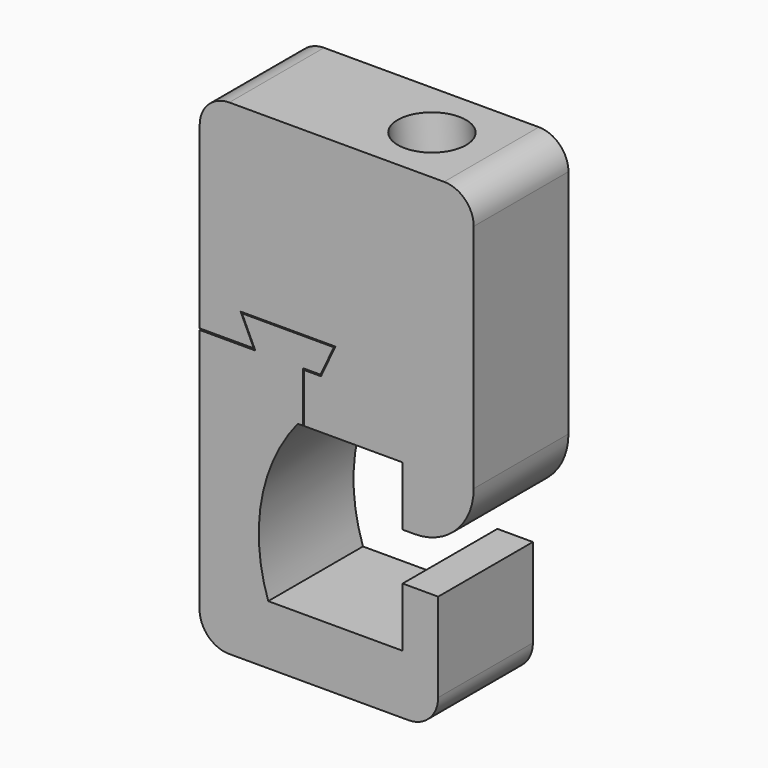
from build123d import *

# Parameters (mm, degrees)
F2_DEPTH = 20
F3_DEPTH = 20
F6_R     = 5.75
F7_DEPTH = 45
F8_R     = 5
F9_R     = 10


# Not quite as in the source:
# - ends of sketch curves that miss each other by under 0.0002 mm in the source are joined


with BuildPart() as f2:
    # F0 (on Front) → F2 (new body)
    with BuildSketch(Plane.XZ):
        with BuildLine():
            Line((-17.6743378025, 22.4031258792), (-27.0860093031, 22.4031258792))
            Line((-27.0860093031, 22.4031258792), (-27.0860093031, -19.1468741208))
            ThreePointArc((-27.0860093031, -19.1468741208), (-25.6215432091, -22.6824080268), (-22.0860093031, -24.1468741208))
            Line((-22.0860093031, -24.1468741208), (8.2122150655, -24.1468741208))
            ThreePointArc((8.2122150655, -24.1468741208), (11.7477489715, -22.6824080268), (13.2122150655, -19.1468741208))
            Line((13.2122150655, -19.1468741208), (13.2122150655, -4.1468741208))
            Line((13.2122150655, -4.1468741208), (7.2122150655, -4.1468741208))
            Line((7.2122150655, -4.1468741208), (7.2122150655, -14.1468741208))
            Line((7.2122150655, -14.1468741208), (-15.4877849345, -14.1468741208))
            ThreePointArc((-15.4877849345, -14.1468741208), (-16.633584051, 0.5013324305), (-10.5006873054, 13.8531258792))
            Line((-10.5006873054, 13.8531258792), (-9.6008945616, 13.8531258792))
            Line((-9.6008945616, 13.8531258792), (-9.6008945616, 22.4031258792))
            Line((-9.6008945616, 22.4031258792), (-6.6508978025, 22.4031258792))
            Line((-6.6508978025, 22.4031258792), (-4.4126178025, 27.2031328292))
            Line((-4.4126178025, 27.2031328292), (-19.9126178025, 27.2031328292))
            Line((-19.9126178025, 27.2031328292), (-17.6743378025, 22.4031258792))
        make_face()
    extrude(amount=F2_DEPTH)


with BuildPart() as f3:
    # F1 (on Front) → F3 (new body)
    with BuildSketch(Plane.XZ):
        Polygon((-9.4277657694, 13.8645800784), (7.2156684956, 13.8645800784), (7.2156684956, 3.8645800784), (19.2156684956, 3.8645800784), (19.2156684956, 57.8645800784), (-27.0665612229, 57.8645800784), (-27.0665612229, 22.6542197451), (-17.9396021321, 22.6542197451), (-20.1487108764, 27.3916687354), (-4.1487108764, 27.3916687354), (-6.5764416154, 22.1853833646), (-9.4277657694, 22.1853833646), align=None)
    extrude(amount=F3_DEPTH)

    # F6 (on face) → F7 (cut)
    with BuildSketch(Plane(origin=(-6.1854109913, 0, 70.6995711451), x_dir=(0.9961946981, 0, 0.0871557427), z_dir=(0.0871557427, 0, -0.9961946981))):
        with Locations((9.1857775311, 10)):
            Circle(F6_R)
    extrude(amount=F7_DEPTH, mode=Mode.SUBTRACT)

    # F8
    f8_edges = [f3.edges().sort_by_distance(p)[0] for p in [
        (-27.066561, -10, 57.86458),
        (19.215668, -10, 57.86458),
    ]]
    fillet(f8_edges, radius=F8_R)

    # F9
    f9_edges = [f3.edges().sort_by_distance(p)[0] for p in [
        (19.215668, -10, 3.86458),
    ]]
    fillet(f9_edges, radius=F9_R)


solid = Compound([f2.part, f3.part])
